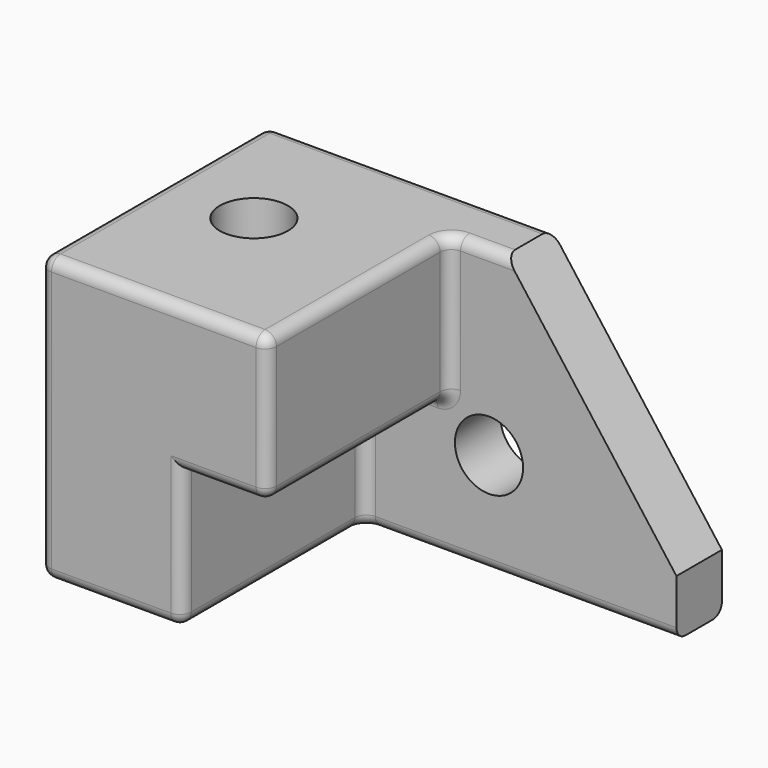
from build123d import *

# Parameters (mm, degrees)
F0_W     = 203.2
F0_H     = 127
F1_DEPTH = 127
F3_DEPTH = 101.6
F4_SIZE2 = 101.6
F4_SIZE  = 76.2
F5_R     = 5.08
F6_R     = 15.24
F7_DEPTH = 1270
F8_R     = 15.24
F9_DEPTH = 12903.2


with BuildPart() as f1:
    # F0 (on Front) → F1 (new body)
    with BuildSketch(Plane.XZ):
        with Locations((20.8130544846, 1.564221409)):
            Rectangle(F0_W, F0_H)
    extrude(amount=F1_DEPTH)

    # F2 (on face) → F3 (cut)
    with BuildSketch(Plane.XZ.offset(127)):
        Polygon((122.4130544846, 65.064221409), (20.8130544846, 65.064221409), (20.8130544846, 0), (-17.2869455154, 0), (-17.2869455154, -61.935778591), (122.4130544846, -61.935778591), align=None)
    extrude(amount=-F3_DEPTH, mode=Mode.SUBTRACT)

    # F4
    f4_edges = [f1.edges().sort_by_distance(p)[0] for p in [
        (122.413054, -12.7, 65.064221),
    ]]
    f4_side = f1.faces().sort_by_distance((-13.053612, -55.033333, 65.064221))[0]
    chamfer(f4_edges, length=F4_SIZE, length2=F4_SIZE2, reference=f4_side)

    # F5
    f5_edges = [f1.edges().sort_by_distance(p)[0] for p in [
        (-29.986946, -127, 65.064221),
        (20.813054, -76.2, 65.064221),
        (20.813054, -25.4, 32.532111),
        (20.813054, -76.2, 0),
        (1.763054, -127, 0),
        (20.813054, -127, 32.532111),
        (-17.286946, -127, -30.967889),
        (-49.036946, -127, -61.935779),
        (-17.286946, -76.2, -61.935779),
        (-17.286946, -25.4, -30.967889),
        (-17.286946, 0, 65.064221),
        (-80.786946, -63.5, 65.064221),
        (-80.786946, -127, 1.564221),
        (-80.786946, -63.5, -61.935779),
        (20.813054, 0, -61.935779),
        (-80.786946, 0, 1.564221),
        (52.563054, -25.4, -61.935779),
        (33.513054, -25.4, 65.064221),
        (1.763054, -25.4, 0),
    ]]
    fillet(f5_edges, radius=F5_R)

    # F6 (on face) → F7 (cut)
    with BuildSketch(Plane.XZ.offset(25.4)):
        with Locations((38.5930544846, -16.215778591)):
            Circle(F6_R)
    extrude(amount=-F7_DEPTH, mode=Mode.SUBTRACT)

    # F8 (on face) → F9 (cut)
    with BuildSketch(Plane.XY.offset(65.064221409)):
        with Locations((-39.8652739823, -58.7147325277)):
            Circle(F8_R)
    extrude(amount=-F9_DEPTH, mode=Mode.SUBTRACT)


solid = f1.part
